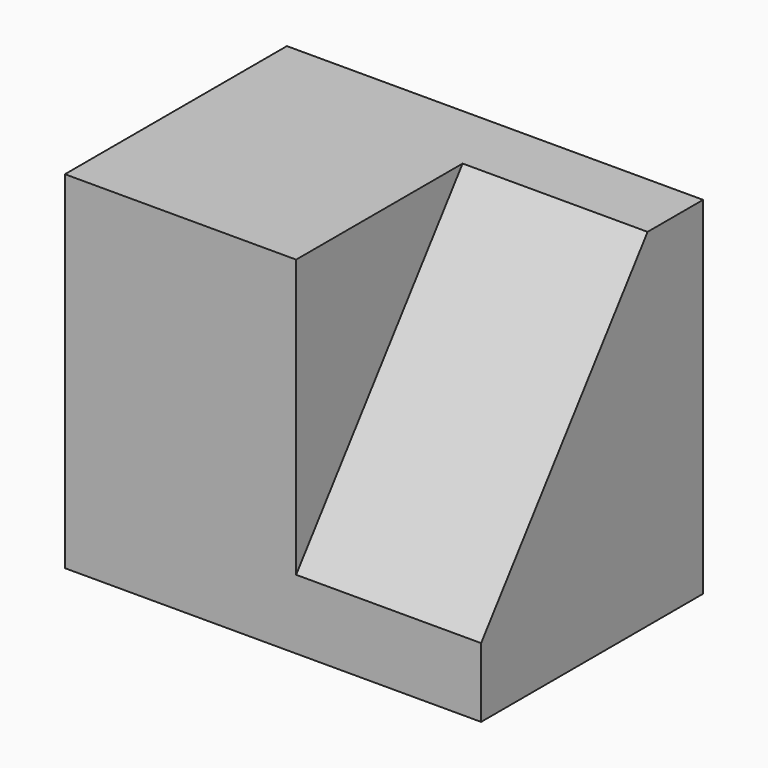
from build123d import *

# Parameters (mm, degrees)
F0_W     = 25.4
F0_H     = 31.75
F1_DEPTH = 38.1
F3_DEPTH = 25.4
F4_DEPTH = 25.4
F6_DEPTH = 16.9333333333


# Not quite as in the source:
# - a length typed as a fraction of an inch, garbled in the dataset ("3 / 203.2 mm" for 3/8 in), is restored


with BuildPart() as f1:
    # F0 (on Right) → F1 (new body)
    with BuildSketch(Plane.YZ):
        with Locations((31.233229906, 15.875)):
            Rectangle(F0_W, F0_H)
    extrude(amount=F1_DEPTH)

    # F2 (on Right) → F3 (cut)
    with BuildSketch(Plane.YZ):
        Polygon((43.7832586467, 31.5612442791), (24.7332586467, 31.5612442791), (44.0856164074, 6.1630439534), align=None)
    extrude(amount=-F3_DEPTH, mode=Mode.SUBTRACT)

    # F2 (on Right) → F4 (cut)
    with BuildSketch(Plane.YZ):
        Polygon((43.7832586467, 31.5612442791), (24.7332586467, 31.5612442791), (44.0856164074, 6.1630439534), align=None)
    extrude(amount=-F4_DEPTH, mode=Mode.SUBTRACT)

    # F5 (on face) → F6 (cut)
    with BuildSketch(Plane.YZ.offset(38.1)):
        Polygon((18.533229906, 6.35), (37.583229906, 31.75), (18.533229906, 31.75), align=None)
    extrude(amount=-F6_DEPTH, mode=Mode.SUBTRACT)


solid = f1.part
